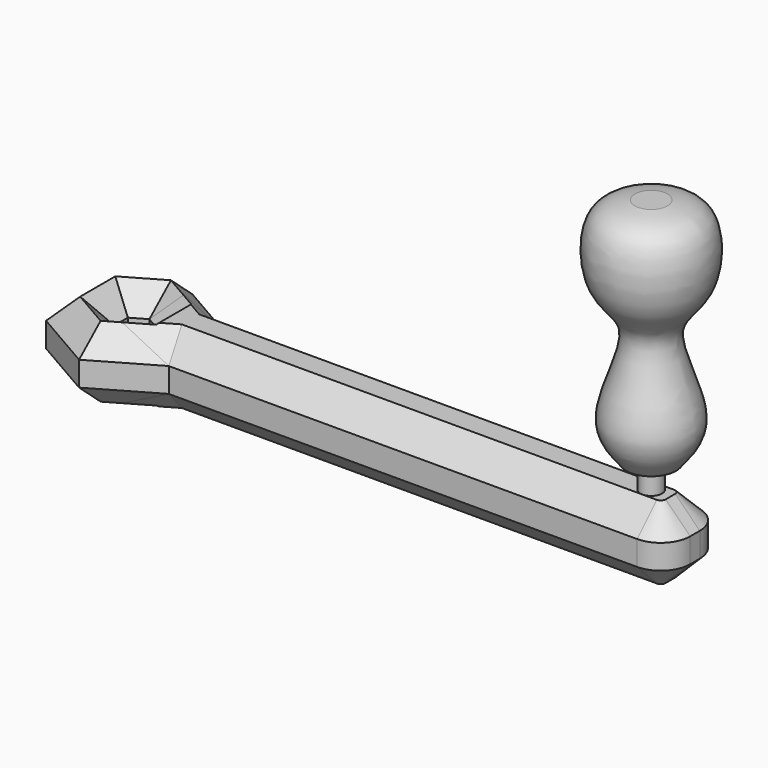
from build123d import *

# Parameters (mm, degrees)
F0_W          = 101.4218062162
F0_H          = 14.4337567297
F1_DEPTH      = 15
F2_R          = 6
F3_T1_DEPTH   = 2.4337567297
F3_T3_DEPTH   = 40.1505866094
F3_T5_DEPTH   = 40.1505866094
F3_T7_DEPTH   = 40.1505866094
F3_T12_DEPTH  = 108.2802211561
F3_T17_DEPTH  = 108.2802211561
F3_T20_ANGLE  = 90
F3_T24_DEPTH  = 40.1505866094
F3_T27_ANGLE  = 90
F3_T31_DEPTH  = 108.2802211561
F3_T36_DEPTH  = 108.2802211561
F3_T41_DEPTH  = 40.1505866094
F3_T46_DEPTH  = 29.1809314948
F3_T52_DEPTH  = 29.1809314948
F3_T58_DEPTH  = 29.1809314948
F3_T64_DEPTH  = 29.1809314948
F3_T70_DEPTH  = 29.1809314948
F3_T76_DEPTH  = 29.1809314948
F3_T82_DEPTH  = 108.2802211561
F3_T87_DEPTH  = 108.2802211561
F3_T90_ANGLE  = 90
F3_T94_DEPTH  = 40.1505866094
F3_T97_ANGLE  = 90
F3_T101_DEPTH = 108.2802211561
F3_T106_DEPTH = 108.2802211561
F3_T111_DEPTH = 40.1505866094
F3_T116_DEPTH = 29.1809314948
F3_T122_DEPTH = 29.1809314948
F3_T128_DEPTH = 29.1809314948
F3_T134_DEPTH = 29.1809314948
F3_T140_DEPTH = 29.1809314948
F3_T146_DEPTH = 29.1809314948
F4_R          = 2.2168783649
F5_DEPTH      = 5


# Not quite as in the source:
# - a fillet or chamfer that OpenCascade refuses, or shapes differently, is made with other operations: its cross-section is extruded or revolved along the edge and cut away or added


with BuildPart() as f1:
    # F0 (on Top) → F1 (new body)
    with BuildSketch(Plane.XY):
        Polygon((12.5, -7.2168783649), (12.5, 7.2168783649), (0, 14.4337567297), (-12.5, 7.2168783649), (-12.5, -7.2168783649), (0, -14.4337567297), align=None)
        Polygon((0, 3.4641016151), (3, 1.7320508076), (3, -1.7320508076), (0, -3.4641016151), (-3, -1.7320508076), (-3, 1.7320508076), align=None, mode=Mode.SUBTRACT)
        with Locations((63.2109031081, 0)):
            Rectangle(F0_W, F0_H)
    extrude(amount=F1_DEPTH)

    # F2
    f2_edges = [f1.edges().sort_by_distance(p)[0] for p in [
        (113.921806, -7.216878, 7.5),
        (113.921806, 7.216878, 7.5),
    ]]
    fillet(f2_edges, radius=F2_R)

    # F3: chamfer of 5 on 32 edges, made by hand

    # F3_s2 → F3_t1 (cut)
    with BuildSketch(Plane.XZ.offset(-1.2168783649)):
        Polygon((108.9218062162, 15), (113.9218062162, 10), (113.9218062162, 15), align=None)
        Polygon((108.9218062162, 0), (113.9218062162, 5), (113.9218062162, 0), align=None)
    extrude(amount=F3_T1_DEPTH, mode=Mode.SUBTRACT)

    # F3_s4 → F3_t3 (cut)
    with BuildSketch(Plane(origin=(-17.3857139903, 10.0376466523, 0), x_dir=(0, 0, 1), z_dir=(0.8660254038, -0.5, 0))):
        Polygon((15, 7.5), (10, 12.5), (15, 12.5), align=None)
        Polygon((0, 7.5), (5, 12.5), (0, 12.5), align=None)
    extrude(amount=F3_T3_DEPTH, mode=Mode.SUBTRACT)

    # F3_s6 → F3_t5 (cut)
    with BuildSketch(Plane.XZ.offset(-20.0752933047)):
        Polygon((-7.5, 15), (-12.5, 10), (-12.5, 15), align=None)
        Polygon((-7.5, 0), (-12.5, 5), (-12.5, 0), align=None)
    extrude(amount=F3_T5_DEPTH, mode=Mode.SUBTRACT)

    # F3_s8 → F3_t7 (cut)
    with BuildSketch(Plane(origin=(17.3857139903, 10.0376466523, 0), x_dir=(0, 0, 1), z_dir=(-0.8660254038, -0.5, 0))):
        Polygon((15, 7.5), (10, 12.5), (15, 12.5), align=None)
        Polygon((0, 7.5), (5, 12.5), (0, 12.5), align=None)
    extrude(amount=F3_T7_DEPTH, mode=Mode.SUBTRACT)


with BuildPart() as f3_tool10:
    # F3_s11 → F3_t12 (new body)
    with BuildSketch(Plane.YZ.offset(-0.3584149398)):
        Polygon((-7.2168783649, 10), (-2.2168783649, 15), (-7.2168783649, 15), align=None)
    extrude(amount=F3_T12_DEPTH)

    split(bisect_by=Plane(origin=(1.5, -2.5980762114, 0), x_dir=(0, 0, 1), z_dir=(-0.5, 0.8660254038, 0)), keep=Keep.TOP)


with BuildPart() as f1_1:
    add(f1.part)

    # F3_t9: cut F3_tool10
    add(f3_tool10.part, mode=Mode.SUBTRACT)


with BuildPart() as f3_tool15:
    # F3_s16 → F3_t17 (new body)
    with BuildSketch(Plane.YZ.offset(-0.3584149398)):
        Polygon((-7.2168783649, 10), (-2.2168783649, 15), (-7.2168783649, 15), align=None)
    extrude(amount=F3_T17_DEPTH)

    split(bisect_by=Plane(origin=(5.625, -9.7427857926, 11.25), x_dir=(0.8660254038, 0.5, 0), z_dir=(0.3535533906, -0.6123724357, 0.7071067812)), keep=Keep.TOP)


with BuildPart() as f1_2:
    add(f1_1.part)

    # F3_t14: cut F3_tool15
    add(f3_tool15.part, mode=Mode.SUBTRACT)

    # F3_s19 → F3_t20 (revolve, cut)
    with BuildSketch(Plane.YZ.offset(107.9218062162)):
        Polygon((-7.2168783649, 10), (-2.2168783649, 15), (-7.2168783649, 15), align=None)
    revolve(axis=Axis((107.9218062162, -1.2168783649, 15), (0, 0, 1)), revolution_arc=F3_T20_ANGLE, mode=Mode.SUBTRACT)


with BuildPart() as f3_tool22:
    # F3_s23 → F3_t24 (new body)
    with BuildSketch(Plane(origin=(-17.3857139903, -10.0376466523, 0), x_dir=(0, 0, 1), z_dir=(0.8660254038, 0.5, 0))):
        Polygon((10, 12.5), (15, 7.5), (15, 12.5), align=None)
    extrude(amount=F3_T24_DEPTH)

    split(bisect_by=Plane(origin=(0, -8.6084391824, 8.6084391824), x_dir=(1, 0, 0), z_dir=(0, -0.7071067812, 0.7071067812)), keep=Keep.TOP)


with BuildPart() as f1_3:
    add(f1_2.part)

    # F3_t21: cut F3_tool22
    add(f3_tool22.part, mode=Mode.SUBTRACT)

    # F3_s26 → F3_t27 (revolve, cut)
    with BuildSketch(Plane.XZ.offset(-1.2168783649)):
        Polygon((108.9218062162, 15), (113.9218062162, 10), (113.9218062162, 15), align=None)
    revolve(axis=Axis((107.9218062162, 1.2168783649, 15), (0, 0, 1)), revolution_arc=F3_T27_ANGLE, mode=Mode.SUBTRACT)


with BuildPart() as f3_tool29:
    # F3_s30 → F3_t31 (new body)
    with BuildSketch(Plane.YZ.offset(107.9218062162)):
        Polygon((2.2168783649, 15), (7.2168783649, 10), (7.2168783649, 15), align=None)
    extrude(amount=-F3_T31_DEPTH)

    split(bisect_by=Plane(origin=(5.625, 9.7427857926, 11.25), x_dir=(-0.8660254038, 0.5, 0), z_dir=(0.3535533906, 0.6123724357, 0.7071067812)), keep=Keep.TOP)


with BuildPart() as f1_4:
    add(f1_3.part)

    # F3_t28: cut F3_tool29
    add(f3_tool29.part, mode=Mode.SUBTRACT)


with BuildPart() as f3_tool34:
    # F3_s35 → F3_t36 (new body)
    with BuildSketch(Plane.YZ.offset(107.9218062162)):
        Polygon((2.2168783649, 15), (7.2168783649, 10), (7.2168783649, 15), align=None)
    extrude(amount=-F3_T36_DEPTH)

    split(bisect_by=Plane(origin=(1.5, 2.5980762114, 0), x_dir=(0, 0, 1), z_dir=(-0.5, -0.8660254038, 0)), keep=Keep.TOP)


with BuildPart() as f1_5:
    add(f1_4.part)

    # F3_t33: cut F3_tool34
    add(f3_tool34.part, mode=Mode.SUBTRACT)


with BuildPart() as f3_tool39:
    # F3_s40 → F3_t41 (new body)
    with BuildSketch(Plane(origin=(17.3857139903, -10.0376466523, 0), x_dir=(0, 0, 1), z_dir=(-0.8660254038, 0.5, 0))):
        Polygon((15, 7.5), (10, 12.5), (15, 12.5), align=None)
    extrude(amount=F3_T41_DEPTH)

    split(bisect_by=Plane(origin=(0, 8.6084391824, 8.6084391824), x_dir=(1, 0, 0), z_dir=(0, 0.7071067812, 0.7071067812)), keep=Keep.TOP)


with BuildPart() as f1_6:
    add(f1_5.part)

    # F3_t38: cut F3_tool39
    add(f3_tool39.part, mode=Mode.SUBTRACT)


with BuildPart() as f3_tool44:
    # F3_s45 → F3_t46 (new body)
    with BuildSketch(Plane(origin=(-12.6357139903, -7.2952328737, 0), x_dir=(0, 0, 1), z_dir=(0.8660254038, 0.5, 0))):
        Polygon((15, -8), (10, -3), (15, -3), align=None)
    extrude(amount=F3_T46_DEPTH)

    split(bisect_by=Plane(origin=(3.5, 0, 3.5), x_dir=(0, 1, 0), z_dir=(0.7071067812, 0, 0.7071067812)), keep=Keep.TOP)

    split(bisect_by=Plane(origin=(-1.75, -3.0310889132, 3.5), x_dir=(0.8660254038, -0.5, 0), z_dir=(-0.3535533906, -0.6123724357, 0.7071067812)), keep=Keep.TOP)


with BuildPart() as f1_7:
    add(f1_6.part)

    # F3_t43: cut F3_tool44
    add(f3_tool44.part, mode=Mode.SUBTRACT)


with BuildPart() as f3_tool50:
    # F3_s51 → F3_t52 (new body)
    with BuildSketch(Plane(origin=(-12.6357139903, 7.2952328737, 0), x_dir=(0, 0, 1), z_dir=(0.8660254038, -0.5, 0))):
        Polygon((15, -8), (10, -3), (15, -3), align=None)
    extrude(amount=F3_T52_DEPTH)

    split(bisect_by=Plane(origin=(-3.5, 0, 3.5), x_dir=(0, 1, 0), z_dir=(-0.7071067812, 0, 0.7071067812)), keep=Keep.TOP)

    split(bisect_by=Plane(origin=(1.75, -3.0310889132, 3.5), x_dir=(0.8660254038, 0.5, 0), z_dir=(0.3535533906, -0.6123724357, 0.7071067812)), keep=Keep.TOP)


with BuildPart() as f1_8:
    add(f1_7.part)

    # F3_t49: cut F3_tool50
    add(f3_tool50.part, mode=Mode.SUBTRACT)


with BuildPart() as f3_tool56:
    # F3_s57 → F3_t58 (new body)
    with BuildSketch(Plane.XZ.offset(-14.5904657474)):
        Polygon((8, 15), (3, 10), (3, 15), align=None)
    extrude(amount=F3_T58_DEPTH)

    split(bisect_by=Plane(origin=(-1.75, 3.0310889132, 3.5), x_dir=(-0.8660254038, -0.5, 0), z_dir=(-0.3535533906, 0.6123724357, 0.7071067812)), keep=Keep.TOP)

    split(bisect_by=Plane(origin=(-1.75, -3.0310889132, 3.5), x_dir=(0.8660254038, -0.5, 0), z_dir=(-0.3535533906, -0.6123724357, 0.7071067812)), keep=Keep.TOP)


with BuildPart() as f1_9:
    add(f1_8.part)

    # F3_t55: cut F3_tool56
    add(f3_tool56.part, mode=Mode.SUBTRACT)


with BuildPart() as f3_tool62:
    # F3_s63 → F3_t64 (new body)
    with BuildSketch(Plane(origin=(12.6357139903, 7.2952328737, 0), x_dir=(0, 0, 1), z_dir=(-0.8660254038, -0.5, 0))):
        Polygon((15, -8), (10, -3), (15, -3), align=None)
    extrude(amount=F3_T64_DEPTH)

    split(bisect_by=Plane(origin=(-3.5, 0, 3.5), x_dir=(0, 1, 0), z_dir=(-0.7071067812, 0, 0.7071067812)), keep=Keep.TOP)

    split(bisect_by=Plane(origin=(1.75, 3.0310889132, 3.5), x_dir=(-0.8660254038, 0.5, 0), z_dir=(0.3535533906, 0.6123724357, 0.7071067812)), keep=Keep.TOP)


with BuildPart() as f1_10:
    add(f1_9.part)

    # F3_t61: cut F3_tool62
    add(f3_tool62.part, mode=Mode.SUBTRACT)


with BuildPart() as f3_tool68:
    # F3_s69 → F3_t70 (new body)
    with BuildSketch(Plane(origin=(12.6357139903, -7.2952328737, 0), x_dir=(0, 0, 1), z_dir=(-0.8660254038, 0.5, 0))):
        Polygon((15, -8), (10, -3), (15, -3), align=None)
    extrude(amount=F3_T70_DEPTH)

    split(bisect_by=Plane(origin=(-1.75, 3.0310889132, 3.5), x_dir=(-0.8660254038, -0.5, 0), z_dir=(-0.3535533906, 0.6123724357, 0.7071067812)), keep=Keep.TOP)

    split(bisect_by=Plane(origin=(3.5, 0, 3.5), x_dir=(0, 1, 0), z_dir=(0.7071067812, 0, 0.7071067812)), keep=Keep.TOP)


with BuildPart() as f1_11:
    add(f1_10.part)

    # F3_t67: cut F3_tool68
    add(f3_tool68.part, mode=Mode.SUBTRACT)


with BuildPart() as f3_tool74:
    # F3_s75 → F3_t76 (new body)
    with BuildSketch(Plane.XZ.offset(14.5904657474)):
        Polygon((-8, 15), (-3, 10), (-3, 15), align=None)
    extrude(amount=-F3_T76_DEPTH)

    split(bisect_by=Plane(origin=(1.75, 3.0310889132, 3.5), x_dir=(-0.8660254038, 0.5, 0), z_dir=(0.3535533906, 0.6123724357, 0.7071067812)), keep=Keep.TOP)

    split(bisect_by=Plane(origin=(1.75, -3.0310889132, 3.5), x_dir=(0.8660254038, 0.5, 0), z_dir=(0.3535533906, -0.6123724357, 0.7071067812)), keep=Keep.TOP)


with BuildPart() as f1_12:
    add(f1_11.part)

    # F3_t73: cut F3_tool74
    add(f3_tool74.part, mode=Mode.SUBTRACT)


with BuildPart() as f3_tool80:
    # F3_s81 → F3_t82 (new body)
    with BuildSketch(Plane.YZ.offset(-0.3584149398)):
        Polygon((-7.2168783649, 5), (-2.2168783649, 0), (-7.2168783649, 0), align=None)
    extrude(amount=F3_T82_DEPTH)

    split(bisect_by=Plane(origin=(1.5, -2.5980762114, 0), x_dir=(0, 0, 1), z_dir=(-0.5, 0.8660254038, 0)), keep=Keep.TOP)


with BuildPart() as f1_13:
    add(f1_12.part)

    # F3_t79: cut F3_tool80
    add(f3_tool80.part, mode=Mode.SUBTRACT)


with BuildPart() as f3_tool85:
    # F3_s86 → F3_t87 (new body)
    with BuildSketch(Plane.YZ.offset(-0.3584149398)):
        Polygon((-7.2168783649, 5), (-2.2168783649, 0), (-7.2168783649, 0), align=None)
    extrude(amount=F3_T87_DEPTH)

    split(bisect_by=Plane(origin=(1.875, -3.2475952642, -3.75), x_dir=(0.8660254038, 0.5, 0), z_dir=(0.3535533906, -0.6123724357, -0.7071067812)), keep=Keep.TOP)


with BuildPart() as f1_14:
    add(f1_13.part)

    # F3_t84: cut F3_tool85
    add(f3_tool85.part, mode=Mode.SUBTRACT)

    # F3_s89 → F3_t90 (revolve, cut)
    with BuildSketch(Plane.YZ.offset(107.9218062162)):
        Polygon((-2.2168783649, 0), (-7.2168783649, 5), (-7.2168783649, 0), align=None)
    revolve(axis=Axis((107.9218062162, -1.2168783649, 0), (0, 0, 1)), revolution_arc=F3_T90_ANGLE, mode=Mode.SUBTRACT)


with BuildPart() as f3_tool92:
    # F3_s93 → F3_t94 (new body)
    with BuildSketch(Plane(origin=(-17.3857139903, -10.0376466523, 0), x_dir=(0, 0, 1), z_dir=(0.8660254038, 0.5, 0))):
        Polygon((0, 7.5), (5, 12.5), (0, 12.5), align=None)
    extrude(amount=F3_T94_DEPTH)

    split(bisect_by=Plane(origin=(0, -1.1084391824, -1.1084391824), x_dir=(1, 0, 0), z_dir=(0, -0.7071067812, -0.7071067812)), keep=Keep.TOP)


with BuildPart() as f1_15:
    add(f1_14.part)

    # F3_t91: cut F3_tool92
    add(f3_tool92.part, mode=Mode.SUBTRACT)

    # F3_s96 → F3_t97 (revolve, cut)
    with BuildSketch(Plane.XZ.offset(-1.2168783649)):
        Polygon((108.9218062162, 0), (113.9218062162, 5), (113.9218062162, 0), align=None)
    revolve(axis=Axis((107.9218062162, 1.2168783649, 0), (0, 0, 1)), revolution_arc=F3_T97_ANGLE, mode=Mode.SUBTRACT)


with BuildPart() as f3_tool99:
    # F3_s100 → F3_t101 (new body)
    with BuildSketch(Plane.YZ.offset(107.9218062162)):
        Polygon((2.2168783649, 0), (7.2168783649, 5), (7.2168783649, 0), align=None)
    extrude(amount=-F3_T101_DEPTH)

    split(bisect_by=Plane(origin=(1.875, 3.2475952642, -3.75), x_dir=(-0.8660254038, 0.5, 0), z_dir=(0.3535533906, 0.6123724357, -0.7071067812)), keep=Keep.TOP)


with BuildPart() as f1_16:
    add(f1_15.part)

    # F3_t98: cut F3_tool99
    add(f3_tool99.part, mode=Mode.SUBTRACT)


with BuildPart() as f3_tool104:
    # F3_s105 → F3_t106 (new body)
    with BuildSketch(Plane.YZ.offset(107.9218062162)):
        Polygon((2.2168783649, 0), (7.2168783649, 5), (7.2168783649, 0), align=None)
    extrude(amount=-F3_T106_DEPTH)

    split(bisect_by=Plane(origin=(1.5, 2.5980762114, 0), x_dir=(0, 0, 1), z_dir=(-0.5, -0.8660254038, 0)), keep=Keep.TOP)


with BuildPart() as f1_17:
    add(f1_16.part)

    # F3_t103: cut F3_tool104
    add(f3_tool104.part, mode=Mode.SUBTRACT)


with BuildPart() as f3_tool109:
    # F3_s110 → F3_t111 (new body)
    with BuildSketch(Plane(origin=(17.3857139903, -10.0376466523, 0), x_dir=(0, 0, 1), z_dir=(-0.8660254038, 0.5, 0))):
        Polygon((0, 7.5), (5, 12.5), (0, 12.5), align=None)
    extrude(amount=F3_T111_DEPTH)

    split(bisect_by=Plane(origin=(0, 1.1084391824, -1.1084391824), x_dir=(1, 0, 0), z_dir=(0, 0.7071067812, -0.7071067812)), keep=Keep.TOP)


with BuildPart() as f1_18:
    add(f1_17.part)

    # F3_t108: cut F3_tool109
    add(f3_tool109.part, mode=Mode.SUBTRACT)


with BuildPart() as f3_tool114:
    # F3_s115 → F3_t116 (new body)
    with BuildSketch(Plane(origin=(-12.6357139903, -7.2952328737, 0), x_dir=(0, 0, 1), z_dir=(0.8660254038, 0.5, 0))):
        Polygon((0, -8), (5, -3), (0, -3), align=None)
    extrude(amount=F3_T116_DEPTH)

    split(bisect_by=Plane(origin=(-4, 0, 4), x_dir=(0, 1, 0), z_dir=(0.7071067812, 0, -0.7071067812)), keep=Keep.TOP)

    split(bisect_by=Plane(origin=(2, 3.4641016151, 4), x_dir=(0.8660254038, -0.5, 0), z_dir=(-0.3535533906, -0.6123724357, -0.7071067812)), keep=Keep.TOP)


with BuildPart() as f1_19:
    add(f1_18.part)

    # F3_t113: cut F3_tool114
    add(f3_tool114.part, mode=Mode.SUBTRACT)


with BuildPart() as f3_tool120:
    # F3_s121 → F3_t122 (new body)
    with BuildSketch(Plane(origin=(-12.6357139903, 7.2952328737, 0), x_dir=(0, 0, 1), z_dir=(0.8660254038, -0.5, 0))):
        Polygon((0, -8), (5, -3), (0, -3), align=None)
    extrude(amount=F3_T122_DEPTH)

    split(bisect_by=Plane(origin=(-2, 3.4641016151, 4), x_dir=(0.8660254038, 0.5, 0), z_dir=(0.3535533906, -0.6123724357, -0.7071067812)), keep=Keep.TOP)

    split(bisect_by=Plane(origin=(4, 0, 4), x_dir=(0, 1, 0), z_dir=(-0.7071067812, 0, -0.7071067812)), keep=Keep.TOP)


with BuildPart() as f1_20:
    add(f1_19.part)

    # F3_t119: cut F3_tool120
    add(f3_tool120.part, mode=Mode.SUBTRACT)


with BuildPart() as f3_tool126:
    # F3_s127 → F3_t128 (new body)
    with BuildSketch(Plane.XZ.offset(-14.5904657474)):
        Polygon((8, 0), (3, 5), (3, 0), align=None)
    extrude(amount=F3_T128_DEPTH)

    split(bisect_by=Plane(origin=(2, -3.4641016151, 4), x_dir=(-0.8660254038, -0.5, 0), z_dir=(-0.3535533906, 0.6123724357, -0.7071067812)), keep=Keep.TOP)

    split(bisect_by=Plane(origin=(2, 3.4641016151, 4), x_dir=(0.8660254038, -0.5, 0), z_dir=(-0.3535533906, -0.6123724357, -0.7071067812)), keep=Keep.TOP)


with BuildPart() as f1_21:
    add(f1_20.part)

    # F3_t125: cut F3_tool126
    add(f3_tool126.part, mode=Mode.SUBTRACT)


with BuildPart() as f3_tool132:
    # F3_s133 → F3_t134 (new body)
    with BuildSketch(Plane(origin=(12.6357139903, 7.2952328737, 0), x_dir=(0, 0, 1), z_dir=(-0.8660254038, -0.5, 0))):
        Polygon((0, -8), (5, -3), (0, -3), align=None)
    extrude(amount=F3_T134_DEPTH)

    split(bisect_by=Plane(origin=(-2, -3.4641016151, 4), x_dir=(-0.8660254038, 0.5, 0), z_dir=(0.3535533906, 0.6123724357, -0.7071067812)), keep=Keep.TOP)

    split(bisect_by=Plane(origin=(4, 0, 4), x_dir=(0, 1, 0), z_dir=(-0.7071067812, 0, -0.7071067812)), keep=Keep.TOP)


with BuildPart() as f1_22:
    add(f1_21.part)

    # F3_t131: cut F3_tool132
    add(f3_tool132.part, mode=Mode.SUBTRACT)


with BuildPart() as f3_tool138:
    # F3_s139 → F3_t140 (new body)
    with BuildSketch(Plane(origin=(12.6357139903, -7.2952328737, 0), x_dir=(0, 0, 1), z_dir=(-0.8660254038, 0.5, 0))):
        Polygon((0, -8), (5, -3), (0, -3), align=None)
    extrude(amount=F3_T140_DEPTH)

    split(bisect_by=Plane(origin=(2, -3.4641016151, 4), x_dir=(-0.8660254038, -0.5, 0), z_dir=(-0.3535533906, 0.6123724357, -0.7071067812)), keep=Keep.TOP)

    split(bisect_by=Plane(origin=(-4, 0, 4), x_dir=(0, 1, 0), z_dir=(0.7071067812, 0, -0.7071067812)), keep=Keep.TOP)


with BuildPart() as f1_23:
    add(f1_22.part)

    # F3_t137: cut F3_tool138
    add(f3_tool138.part, mode=Mode.SUBTRACT)


with BuildPart() as f3_tool144:
    # F3_s145 → F3_t146 (new body)
    with BuildSketch(Plane.XZ.offset(14.5904657474)):
        Polygon((-8, 0), (-3, 5), (-3, 0), align=None)
    extrude(amount=-F3_T146_DEPTH)

    split(bisect_by=Plane(origin=(-2, -3.4641016151, 4), x_dir=(-0.8660254038, 0.5, 0), z_dir=(0.3535533906, 0.6123724357, -0.7071067812)), keep=Keep.TOP)

    split(bisect_by=Plane(origin=(-2, 3.4641016151, 4), x_dir=(0.8660254038, 0.5, 0), z_dir=(0.3535533906, -0.6123724357, -0.7071067812)), keep=Keep.TOP)


with BuildPart() as f1_24:
    add(f1_23.part)

    # F3_t143: cut F3_tool144
    add(f3_tool144.part, mode=Mode.SUBTRACT)

    # F4 (on face) → F5 (join)
    with BuildSketch(Plane.XY.offset(15)):
        with Locations((105, 0)):
            Circle(F4_R)
    extrude(amount=F5_DEPTH)

    # F6 (on Front) → F7 (revolve)
    with BuildSketch(Plane.XZ):
        with BuildLine():
            Line((108.3080768585, 66.9323056936), (105, 66.9323056936))
            Line((105, 66.9323056936), (105, 20))
            Line((105, 20), (110.0828945637, 20))
            add(Edge.make_bspline(
                [(110.0828945637, 20), (112.0426276757, 22.363673848), (116.5861959485, 27.8437592299), (106.6734024331, 44.5470793569), (116.570655373, 49.9594893214), (116.8964211839, 65.5898079545), (110.8957227351, 66.5278041763), (108.3080768585, 66.9323056936)],
                knots=[0, 0, 0, 0, 0.1852557032, 0.4295082555, 0.6154016859, 0.8341515178, 1, 1, 1, 1], degree=3))
        make_face()
    revolve(axis=Axis((105, 0, 43.4661528468), (0, 0, -1)))


solid = f1_24.part
